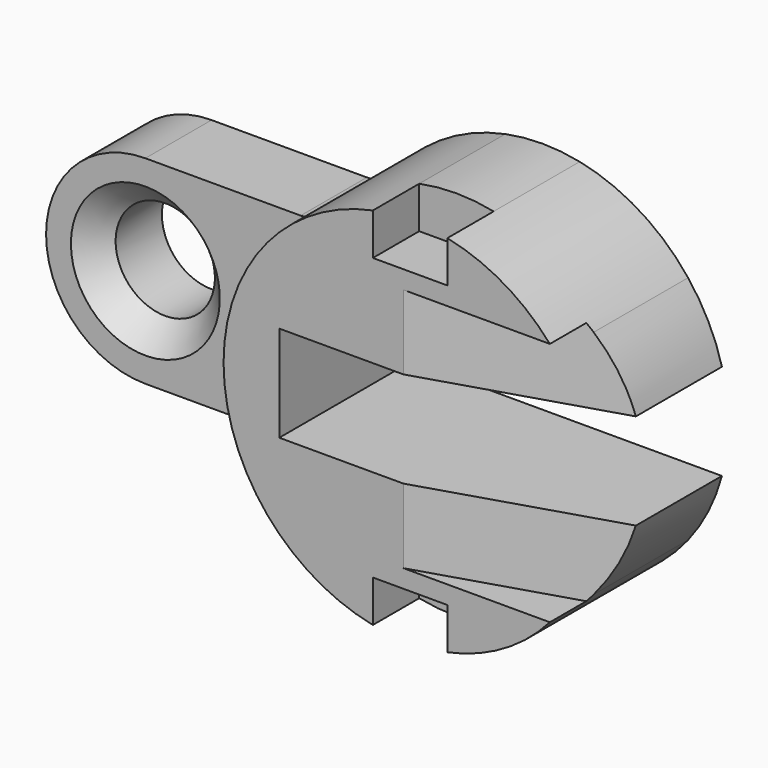
from build123d import *

# Parameters (mm, degrees)
F1_DEPTH = 10
F2_SIZE2 = 3
F2_SIZE  = 3
F3_DEPTH = 20
F4_DEPTH = 13
F6_DEPTH = 9
F8_DEPTH = 9


# Not quite as in the source:
# - after a boolean that leaves OpenCascade's solid faulty, fix() repairs it


with BuildPart() as f1:
    # F0 (on Front) → F1 (new body)
    with BuildSketch(Plane.XZ):
        with BuildLine():
            ThreePointArc((-12.5, 12), (-20.9852813742, 8.4852813742), (-24.5, 0))
            ThreePointArc((-24.5, 0), (-20.9852813742, -8.4852813742), (-12.5, -12))
            Line((-12.5, -12), (6.2676198227, -12))
            ThreePointArc((6.2676198227, -12), (7.6484176342, -12.1944409895), (8.9218219686, -12.7626410385))
            ThreePointArc((8.9218219686, -12.7626410385), (5.9673160107, -6.6829078481), (4.9519324303, 0))
            ThreePointArc((4.9519324303, 0), (5.9673160107, 6.6829078481), (8.9218219686, 12.7626410385))
            ThreePointArc((8.9218219686, 12.7626410385), (7.6484176342, 12.1944409895), (6.2676198227, 12))
            Line((6.2676198227, 12), (-12.5, 12))
        make_face()
        with BuildLine():
            ThreePointArc((-3.5, 0), (-12.5, -9), (-21.5, 0))
            ThreePointArc((-21.5, 0), (-12.5, 9), (-3.5, 0))
        make_face(mode=Mode.SUBTRACT)
        with BuildLine():
            ThreePointArc((-3.5, 0), (-12.5, 9), (-21.5, 0))
            ThreePointArc((-21.5, 0), (-12.5, -9), (-3.5, 0))
        make_face()
        with BuildLine():
            ThreePointArc((-6.5, 0), (-12.5, -6), (-18.5, 0))
            ThreePointArc((-18.5, 0), (-12.5, 6), (-6.5, 0))
        make_face(mode=Mode.SUBTRACT)
    extrude(amount=F1_DEPTH)

    # F2
    f2_edges = [f1.edges().sort_by_distance(p)[0] for p in [
        (-6.5, -10, 0),
    ]]
    chamfer(f2_edges, length=F2_SIZE, length2=F2_SIZE2)

    # F0 (on Front) → F3 (join)
    with BuildSketch(Plane.XZ):
        with BuildLine():
            ThreePointArc((4.9519324303, 0), (5.9673160107, -6.6829078481), (8.9218219686, -12.7626410385))
            ThreePointArc((8.9218219686, -12.7626410385), (15.0571220775, -18.7781435802), (23, -22.0551648744))
            Line((23, -22.0551648744), (23, -17))
            Line((23, -17), (27.5, -17))
            Line((27.5, -17), (32, -17))
            Line((32, -17), (32, -22.0355413226))
            ThreePointArc((32, -22.0355413226), (39.2642294703, -19.1499252907), (45.1029145419, -13.9532372766))
            Line((45.1029145419, -13.9532372766), (27.4519324303, -13.9532372766))
            Line((27.4519324303, -13.9532372766), (27.4519324303, -5.8079371229))
            Line((27.4519324303, -5.8079371229), (11.6894085114, -5.8079371229))
            Line((11.6894085114, -5.8079371229), (11.6894085114, 0))
            Line((11.6894085114, 0), (11.6894085114, 5.8079371229))
            Line((11.6894085114, 5.8079371229), (27.5485839971, 5.8079371229))
            Line((27.5485839971, 5.8079371229), (27.4519324303, 13.9532372766))
            Line((27.4519324303, 13.9532372766), (45.1029145419, 13.9532372766))
            ThreePointArc((45.1029145419, 13.9532372766), (39.2642294703, 19.1499252907), (32, 22.0355413226))
            Line((32, 22.0355413226), (32, 17))
            Line((32, 17), (27.5, 17))
            Line((27.5, 17), (23, 17))
            Line((23, 17), (23, 22.0551648744))
            ThreePointArc((23, 22.0551648744), (15.0571220775, 18.7781435802), (8.9218219686, 12.7626410385))
            ThreePointArc((8.9218219686, 12.7626410385), (5.9673160107, 6.6829078481), (4.9519324303, 0))
        make_face()
        with BuildLine():
            ThreePointArc((49.1894085114, 5.8079371229), (47.562853303, 10.0896413044), (45.1029145419, 13.9532372766))
            Line((45.1029145419, 13.9532372766), (27.4519324303, 13.9532372766))
            Line((27.4519324303, 13.9532372766), (27.5485839971, 5.8079371229))
            Line((27.5485839971, 5.8079371229), (49.1894085114, 5.8079371229))
        make_face()
        with BuildLine():
            Line((27.4519324303, -13.9532372766), (45.1029145419, -13.9532372766))
            ThreePointArc((45.1029145419, -13.9532372766), (47.562853303, -10.0896413044), (49.1894085114, -5.8079371229))
            Line((49.1894085114, -5.8079371229), (27.4519324303, -5.8079371229))
            Line((27.4519324303, -5.8079371229), (27.4519324303, -13.9532372766))
        make_face()
    extrude(amount=F3_DEPTH)

    # F0 (on Front) → F4 (join)
    with BuildSketch(Plane.XZ):
        with BuildLine():
            ThreePointArc((32, 22.0355413226), (27.5009911931, 22.4999465163), (23, 22.0551648744))
            Line((23, 22.0551648744), (23, 17))
            Line((23, 17), (27.5, 17))
            Line((27.5, 17), (32, 17))
            Line((32, 17), (32, 22.0355413226))
        make_face()
        with BuildLine():
            Line((23, -17), (23, -22.0551648744))
            ThreePointArc((23, -22.0551648744), (27.5009911931, -22.4999465163), (32, -22.0355413226))
            Line((32, -22.0355413226), (32, -17))
            Line((32, -17), (27.5, -17))
            Line((27.5, -17), (23, -17))
        make_face()
    extrude(amount=F4_DEPTH)

    # F5 (on face) → F6 (cut)
    with BuildSketch(Plane(origin=(0, 0, 5.8079371229), x_dir=(1, 0, 0), z_dir=(0, 0, -1))):
        Polygon((49.1894085114, 13), (49.1894085114, 20), (26.6894085114, 20), align=None)
    extrude(amount=-F6_DEPTH, mode=Mode.SUBTRACT)

    # F7 (on face) → F8 (cut)
    with BuildSketch(Plane.XY.offset(-5.8079371229)):
        Polygon((26.6894085114, -20), (49.1894085114, -20), (49.1894085114, -13), align=None)
    extrude(amount=-F8_DEPTH, mode=Mode.SUBTRACT)

    add(f1.part.fix(), mode=Mode.REPLACE)


solid = f1.part
